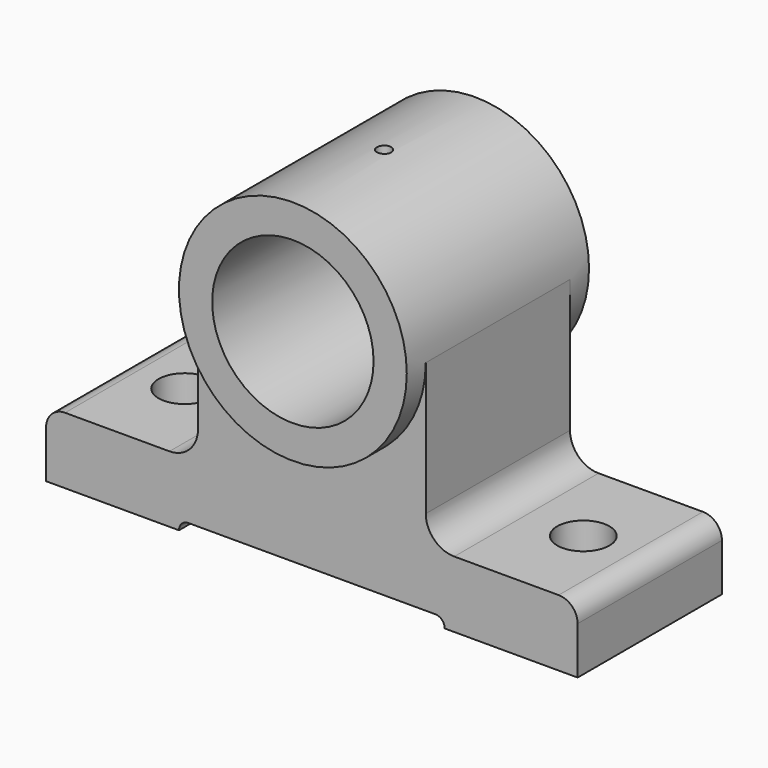
from build123d import *

# Parameters (mm, degrees)
F0_R     = 26.9875
F1_DEPTH = 38.1
F2_DEPTH = 30.1625
F3_R     = 8.73125
F4_DEPTH = 76.201
F5_R     = 2.38125
F6_DEPTH = 38.101
F7_R     = 9.525
F8_R     = 6.35
F9_R     = 3.17499


# Not quite as in the source:
# - a fillet or chamfer is up to 0.001 mm smaller than in the source, because OpenCascade refuses the exact size


with BuildPart() as f1:
    # F0 (on Front) → F1 (new body, symmetric)
    with BuildSketch(Plane.XZ):
        with BuildLine():
            ThreePointArc((-38.1, 0), (0, -38.1), (38.1, 0))
            ThreePointArc((38.1, 0), (0, 38.1), (-38.1, 0))
        make_face()
        Circle(F0_R, mode=Mode.SUBTRACT)
    extrude(amount=F1_DEPTH, both=True)

    # F0 (on Front) → F2 (join, symmetric)
    with BuildSketch(Plane.XZ):
        with BuildLine():
            ThreePointArc((-38.1, 0), (0, -38.1), (38.1, 0))
            ThreePointArc((38.1, 0), (0, 38.1), (-38.1, 0))
        make_face()
        Circle(F0_R, mode=Mode.SUBTRACT)
        with BuildLine():
            Line((38.1, -53.975), (38.1, 0))
            ThreePointArc((38.1, 0), (0, -38.1), (-38.1, 0))
            Line((-38.1, 0), (-38.1, -53.975))
            Line((-38.1, -53.975), (-88.9, -53.975))
            Line((-88.9, -53.975), (-88.9, -76.2))
            Line((-88.9, -76.2), (-44.45, -76.2))
            Line((-44.45, -76.2), (-44.45, -73.025))
            Line((-44.45, -73.025), (0, -73.025))
            Line((0, -73.025), (44.45, -73.025))
            Line((44.45, -73.025), (44.45, -76.2))
            Line((44.45, -76.2), (88.9, -76.2))
            Line((88.9, -76.2), (88.9, -53.975))
            Line((88.9, -53.975), (38.1, -53.975))
        make_face()
    extrude(amount=F2_DEPTH, both=True)

    # F3 (on Top) → F4 (cut, through all)
    with BuildSketch(Plane.XY):
        with Locations((-66.675, 0)):
            Circle(F3_R)
        with Locations((66.675, 0)):
            Circle(F3_R)
    extrude(amount=-F4_DEPTH, mode=Mode.SUBTRACT)

    # F5 (on Top) → F6 (cut, through all)
    with BuildSketch(Plane.XY):
        Circle(F5_R)
    extrude(amount=F6_DEPTH, mode=Mode.SUBTRACT)

    # F7
    f7_edges = [f1.edges().sort_by_distance(p)[0] for p in [
        (38.1, 0, -53.975),
        (-38.1, 0, -53.975),
    ]]
    fillet(f7_edges, radius=F7_R)

    # F8
    f8_edges = [f1.edges().sort_by_distance(p)[0] for p in [
        (-88.9, 0, -53.975),
        (88.9, 0, -53.975),
    ]]
    fillet(f8_edges, radius=F8_R)

    # F9 (radius 3.175 in the source; OpenCascade refuses exactly that, so slightly less here)
    f9_edges = [f1.edges().sort_by_distance(p)[0] for p in [
        (-44.45, 0, -73.025),
        (44.45, 0, -73.025),
    ]]
    fillet(f9_edges, radius=F9_R)


solid = f1.part
